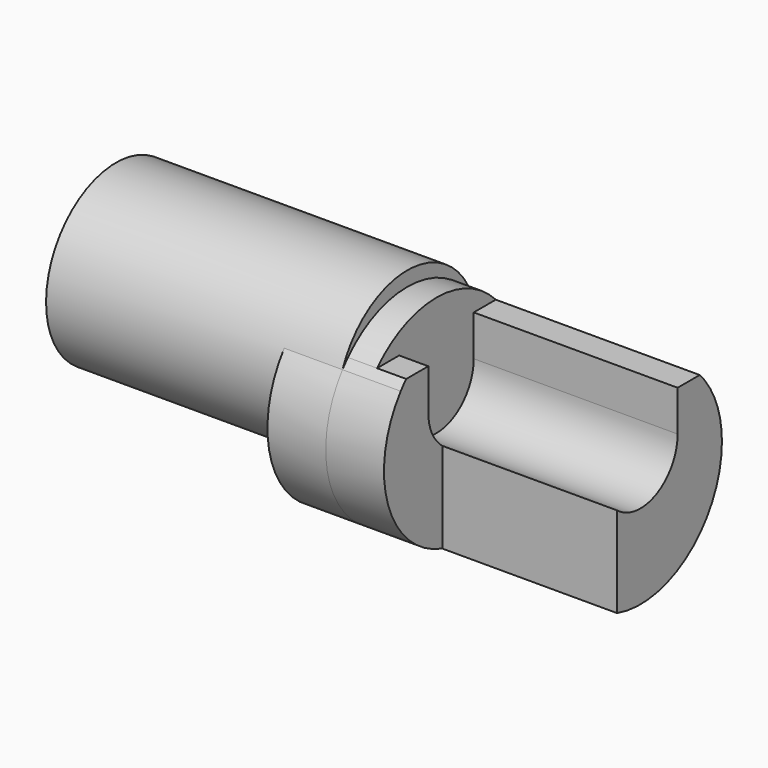
from build123d import *
from build123d import SkipClean  # not in build123d's __all__

# Parameters (mm, degrees)
F1_DEPTH = 40
F2_DEPTH = 50
F3_DEPTH = 10
F4_DEPTH = 5
F5_DEPTH = 10


with BuildPart() as f1:
    # F0 (on Right) → F1 (new body)
    with BuildSketch(Plane.YZ):
        with BuildLine():
            ThreePointArc((50.7187942612, 39.2482171013), (49.7957965967, 44.8565139525), (47.1241664245, 49.8732171013))
            ThreePointArc((47.1241664245, 49.8732171013), (47.9425944237, 47.1134760382), (48.2187942612, 44.2482171013))
            ThreePointArc((48.2187942612, 44.2482171013), (41.8790482991, 32.0007683874), (28.2187942612, 30.1060814776))
            Line((28.2187942612, 30.1060814776), (28.2187942612, 22.4777072701))
            ThreePointArc((28.2187942612, 22.4777072701), (43.6770445929, 25.2170019009), (50.7187942612, 39.2482171013))
        make_face()
        with BuildLine():
            ThreePointArc((47.1241664245, 49.8732171013), (46.5580784274, 50.5757719095), (45.9565334641, 51.2482171013))
            Line((45.9565334641, 51.2482171013), (41.2187942612, 51.2482171013))
            Line((41.2187942612, 51.2482171013), (41.2187942612, 44.2482171013))
            ThreePointArc((41.2187942612, 44.2482171013), (36.6828958764, 37.0371145504), (28.2187942612, 38.0032191029))
            Line((28.2187942612, 38.0032191029), (28.2187942612, 30.1060814776))
            ThreePointArc((28.2187942612, 30.1060814776), (41.8790482991, 32.0007683874), (48.2187942612, 44.2482171013))
            ThreePointArc((48.2187942612, 44.2482171013), (47.9425944237, 47.1134760382), (47.1241664245, 49.8732171013))
        make_face()
    extrude(amount=F1_DEPTH)

    # F0 (on Right) → F2 (join)
    with BuildSketch(Plane.YZ):
        with BuildLine():
            Line((25.2187942612, 51.2482171013), (20.4810550584, 51.2482171013))
            ThreePointArc((20.4810550584, 51.2482171013), (19.879510095, 50.5757719095), (19.3134220979, 49.8732171013))
            ThreePointArc((19.3134220979, 49.8732171013), (19.5426037518, 38.0869012394), (28.2187942612, 30.1060814776))
            Line((28.2187942612, 30.1060814776), (28.2187942612, 38.0032191029))
            ThreePointArc((28.2187942612, 38.0032191029), (26.0076917103, 40.7841154862), (25.2187942612, 44.2482171013))
            Line((25.2187942612, 44.2482171013), (25.2187942612, 51.2482171013))
        make_face()
        with BuildLine():
            ThreePointArc((20.4810550584, 51.2482171013), (33.2187942612, 56.7482171013), (45.9565334641, 51.2482171013))
            ThreePointArc((45.9565334641, 51.2482171013), (46.5580784274, 50.5757719095), (47.1241664245, 49.8732171013))
            ThreePointArc((47.1241664245, 49.8732171013), (33.2187942612, 59.2482171013), (19.3134220979, 49.8732171013))
            ThreePointArc((19.3134220979, 49.8732171013), (19.879510095, 50.5757719095), (20.4810550584, 51.2482171013))
        make_face()
        with BuildLine():
            Line((41.2187942612, 51.2482171013), (45.9565334641, 51.2482171013))
            ThreePointArc((45.9565334641, 51.2482171013), (33.2187942612, 56.7482171013), (20.4810550584, 51.2482171013))
            Line((20.4810550584, 51.2482171013), (25.2187942612, 51.2482171013))
            Line((25.2187942612, 51.2482171013), (25.2187942612, 44.2482171013))
            ThreePointArc((25.2187942612, 44.2482171013), (26.0076917103, 40.7841154862), (28.2187942612, 38.0032191029))
            ThreePointArc((28.2187942612, 38.0032191029), (36.6828958764, 37.0371145504), (41.2187942612, 44.2482171013))
            Line((41.2187942612, 44.2482171013), (41.2187942612, 51.2482171013))
        make_face()
        with BuildLine():
            ThreePointArc((47.1241664245, 49.8732171013), (46.5580784274, 50.5757719095), (45.9565334641, 51.2482171013))
            Line((45.9565334641, 51.2482171013), (41.2187942612, 51.2482171013))
            Line((41.2187942612, 51.2482171013), (41.2187942612, 44.2482171013))
            ThreePointArc((41.2187942612, 44.2482171013), (36.6828958764, 37.0371145504), (28.2187942612, 38.0032191029))
            Line((28.2187942612, 38.0032191029), (28.2187942612, 30.1060814776))
            ThreePointArc((28.2187942612, 30.1060814776), (41.8790482991, 32.0007683874), (48.2187942612, 44.2482171013))
            ThreePointArc((48.2187942612, 44.2482171013), (47.9425944237, 47.1134760382), (47.1241664245, 49.8732171013))
        make_face()
    extrude(amount=-F2_DEPTH)

    # F0 (on Right) → F3 (join)
    with BuildSketch(Plane.YZ):
        with BuildLine():
            Line((25.2187942612, 51.2482171013), (20.4810550584, 51.2482171013))
            ThreePointArc((20.4810550584, 51.2482171013), (19.879510095, 50.5757719095), (19.3134220979, 49.8732171013))
            ThreePointArc((19.3134220979, 49.8732171013), (19.5426037518, 38.0869012394), (28.2187942612, 30.1060814776))
            Line((28.2187942612, 30.1060814776), (28.2187942612, 38.0032191029))
            ThreePointArc((28.2187942612, 38.0032191029), (26.0076917103, 40.7841154862), (25.2187942612, 44.2482171013))
            Line((25.2187942612, 44.2482171013), (25.2187942612, 51.2482171013))
        make_face()
        with BuildLine():
            ThreePointArc((28.2187942612, 30.1060814776), (19.5426037518, 38.0869012394), (19.3134220979, 49.8732171013))
            ThreePointArc((19.3134220979, 49.8732171013), (16.5760251441, 33.8382045215), (28.2187942612, 22.4777072701))
            Line((28.2187942612, 22.4777072701), (28.2187942612, 30.1060814776))
        make_face()
    extrude(amount=F3_DEPTH)

    # F0 (on Right) → F4 (join)
    with BuildSketch(Plane.YZ):
        with BuildLine():
            Line((41.2187942612, 51.2482171013), (45.9565334641, 51.2482171013))
            ThreePointArc((45.9565334641, 51.2482171013), (33.2187942612, 56.7482171013), (20.4810550584, 51.2482171013))
            Line((20.4810550584, 51.2482171013), (25.2187942612, 51.2482171013))
            Line((25.2187942612, 51.2482171013), (25.2187942612, 44.2482171013))
            ThreePointArc((25.2187942612, 44.2482171013), (26.0076917103, 40.7841154862), (28.2187942612, 38.0032191029))
            ThreePointArc((28.2187942612, 38.0032191029), (36.6828958764, 37.0371145504), (41.2187942612, 44.2482171013))
            Line((41.2187942612, 44.2482171013), (41.2187942612, 51.2482171013))
        make_face()
    extrude(amount=F4_DEPTH)

    # F0 (on Right) → F5 (join)
    with BuildSketch(Plane.YZ):
        with BuildLine():
            ThreePointArc((28.2187942612, 30.1060814776), (19.5426037518, 38.0869012394), (19.3134220979, 49.8732171013))
            ThreePointArc((19.3134220979, 49.8732171013), (16.5760251441, 33.8382045215), (28.2187942612, 22.4777072701))
            Line((28.2187942612, 22.4777072701), (28.2187942612, 30.1060814776))
        make_face()
        with BuildLine():
            ThreePointArc((50.7187942612, 39.2482171013), (49.7957965967, 44.8565139525), (47.1241664245, 49.8732171013))
            ThreePointArc((47.1241664245, 49.8732171013), (47.9425944237, 47.1134760382), (48.2187942612, 44.2482171013))
            ThreePointArc((48.2187942612, 44.2482171013), (41.8790482991, 32.0007683874), (28.2187942612, 30.1060814776))
            Line((28.2187942612, 30.1060814776), (28.2187942612, 22.4777072701))
            ThreePointArc((28.2187942612, 22.4777072701), (43.6770445929, 25.2170019009), (50.7187942612, 39.2482171013))
        make_face()
    with SkipClean():  # cleaning this boolean's faces spoils the solid; the shape is the same uncleaned
        extrude(amount=-F5_DEPTH)


solid = f1.part
